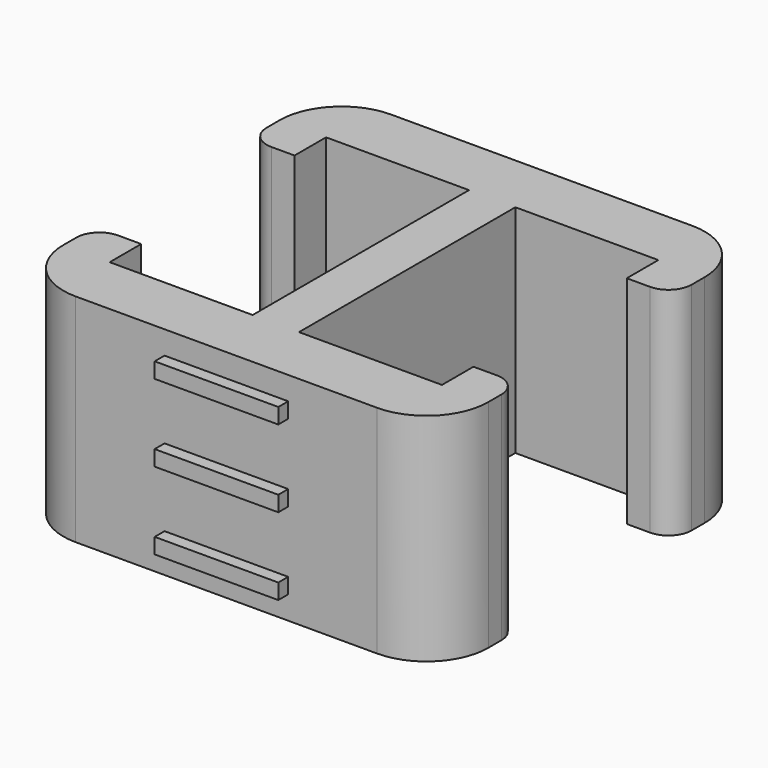
from build123d import *

# Parameters (mm, degrees)
F0_W     = 1.5
F0_H     = 8.75
F1_DEPTH = 7
F2_R     = 0.75
F3_R     = 2
F4_W     = 4
F4_H     = 0.5
F5_DEPTH = 0.4
F6_W     = 4
F6_H     = 0.5
F7_DEPTH = 0.4


# Not quite as in the source:
# - a feature names something its author has since deleted; it is built from what else it names


with BuildPart() as f1:
    # F0 (on Top) → F1 (new body)
    with BuildSketch(Plane.XY):
        Polygon((5.375, -4.375), (0.75, -4.375), (-0.75, -4.375), (-5.375, -4.375), (-5.375, -6.375), (5.375, -6.375), align=None)
        Rectangle(F0_W, F0_H)
        Polygon((-0.75, 4.375), (0.75, 4.375), (5.375, 4.375), (5.375, 6.375), (-5.375, 6.375), (-5.375, 4.375), align=None)
        Polygon((5.375, -3.1), (5.375, -4.375), (5.375, -6.375), (6.875, -6.375), (6.875, -3.1), align=None)
        Polygon((-5.375, -6.375), (-5.375, -4.375), (-5.375, -3.1), (-6.875, -3.1), (-6.875, -6.375), align=None)
        Polygon((5.375, 6.375), (5.375, 4.375), (5.375, 3.1), (6.875, 3.1), (6.875, 6.375), align=None)
        Polygon((-5.375, 3.1), (-5.375, 4.375), (-5.375, 6.375), (-6.875, 6.375), (-6.875, 3.1), align=None)
    extrude(amount=F1_DEPTH)

    # F2
    f2_edges = [f1.edges().sort_by_distance(p)[0] for p in [
        (-6.875, 3.1, 3.5),
        (6.875, 3.1, 3.5),
        (6.875, -3.1, 3.5),
        (-6.875, -3.1, 3.5),
    ]]
    fillet(f2_edges, radius=F2_R)

    # F3
    f3_edges = [f1.edges().sort_by_distance(p)[0] for p in [
        (-6.875, -6.375, 3.5),
        (6.875, -6.375, 3.5),
        (6.875, 6.375, 3.5),
        (-6.875, 6.375, 3.5),
    ]]
    fillet(f3_edges, radius=F3_R)

    # F4 (on face) → F5 (join)
    with BuildSketch(Plane(origin=(0, 6.375, 0), x_dir=(-1, 0, 0), z_dir=(0, 1, 0))):
        with Locations((0, 1)):
            Rectangle(F4_W, F4_H)
        with Locations((0, 3.5)):
            Rectangle(F4_W, F4_H)
        with Locations((0, 6)):
            Rectangle(F4_W, F4_H)
    extrude(amount=F5_DEPTH)

    # F6 (on face) → F7 (join)
    with BuildSketch(Plane.XZ.offset(6.375)):
        with Locations((0, 3.5)):
            Rectangle(F6_W, F6_H)
        with Locations((0, 6)):
            Rectangle(F6_W, F6_H)
        with Locations((0, 1)):
            Rectangle(F6_W, F6_H)
    extrude(amount=F7_DEPTH)


solid = f1.part
